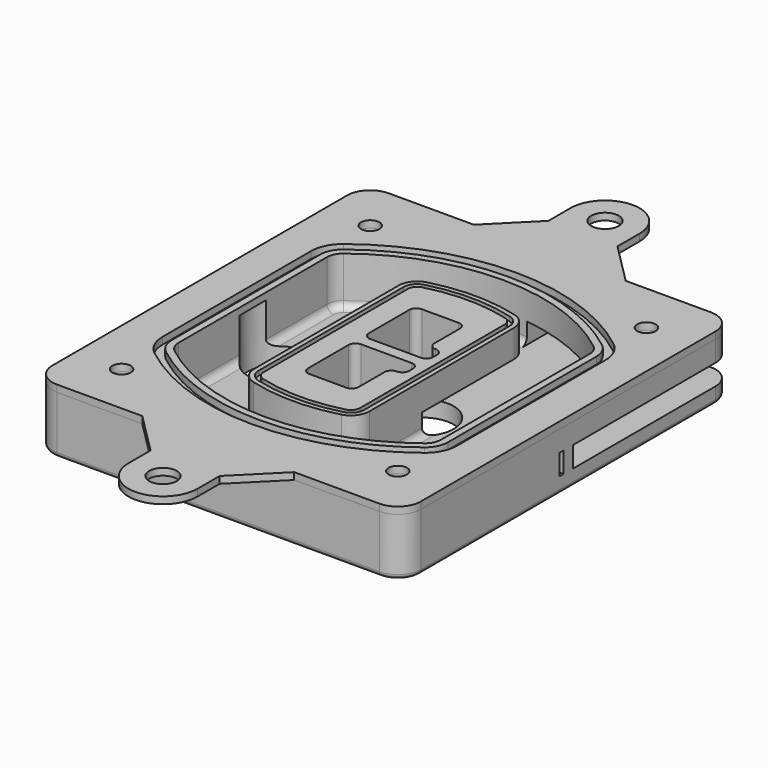
from build123d import *

# Parameters (mm, degrees)
F0_R      = 4
F1_DEPTH  = 25
F2_DEPTH  = 3
F3_DEPTH  = 18
F6_DEPTH  = 21
F7_DEPTH  = 2
F8_DEPTH  = 16
F9_DEPTH  = 25
F4_R      = 6
F4_R_2    = 4
F10_DEPTH = 6
F12_DEPTH = 9
F13_R     = 3
F14_R     = 2
F0_R_2    = 6
F15_DEPTH = 3
F17_DEPTH = 3


with BuildPart() as f1:
    # F0 (on Top) → F1 (new body)
    with BuildSketch(Plane.XY):
        with BuildLine():
            ThreePointArc((-80, -80), (-77.0710678119, -87.0710678119), (-70, -90))
            Line((-70, -90), (-33, -90))
            Line((-33, -90), (33, -90))
            Line((33, -90), (70, -90))
            ThreePointArc((70, -90), (77.0710678119, -87.0710678119), (80, -80))
            Line((80, -80), (80, 80))
            ThreePointArc((80, 80), (77.0710678119, 87.0710678119), (70, 90))
            Line((70, 90), (33, 90))
            Line((33, 90), (-33, 90))
            Line((-33, 90), (-70, 90))
            ThreePointArc((-70, 90), (-77.0710678119, 87.0710678119), (-80, 80))
            Line((-80, 80), (-80, -80))
        make_face()
        with Locations((-60, -67.5)):
            Circle(F0_R, mode=Mode.SUBTRACT)
        with Locations((60, -67.5)):
            Circle(F0_R, mode=Mode.SUBTRACT)
        with Locations((-60, 67.5)):
            Circle(F0_R, mode=Mode.SUBTRACT)
        with BuildLine():
            ThreePointArc((-64, 40.2934422872), (-62.5820384798, 46.4328484224), (-58.6153846154, 51.3286200352))
            ThreePointArc((-58.6153846154, 51.3286200352), (0, 71.5), (58.6153846154, 51.3286200352))
            ThreePointArc((58.6153846154, 51.3286200352), (62.5820384798, 46.4328484224), (64, 40.2934422872))
            Line((64, 40.2934422872), (64, -40.2934422872))
            ThreePointArc((64, -40.2934422872), (62.5820384798, -46.4328484224), (58.6153846154, -51.3286200352))
            ThreePointArc((58.6153846154, -51.3286200352), (0, -71.5), (-58.6153846154, -51.3286200352))
            ThreePointArc((-58.6153846154, -51.3286200352), (-62.5820384798, -46.4328484224), (-64, -40.2934422872))
            Line((-64, -40.2934422872), (-64, 40.2934422872))
        make_face(mode=Mode.SUBTRACT)
        with Locations((60, 67.5)):
            Circle(F0_R, mode=Mode.SUBTRACT)
        with BuildLine():
            ThreePointArc((58.6153846154, 51.3286200352), (0, 71.5), (-58.6153846154, 51.3286200352))
            ThreePointArc((-58.6153846154, 51.3286200352), (-62.5820384798, 46.4328484224), (-64, 40.2934422872))
            Line((-64, 40.2934422872), (-64, -40.2934422872))
            ThreePointArc((-64, -40.2934422872), (-62.5820384798, -46.4328484224), (-58.6153846154, -51.3286200352))
            ThreePointArc((-58.6153846154, -51.3286200352), (0, -71.5), (58.6153846154, -51.3286200352))
            ThreePointArc((58.6153846154, -51.3286200352), (62.5820384798, -46.4328484224), (64, -40.2934422872))
            Line((64, -40.2934422872), (64, 40.2934422872))
            ThreePointArc((64, 40.2934422872), (62.5820384798, 46.4328484224), (58.6153846154, 51.3286200352))
        make_face()
        with BuildLine():
            Line((-60, -40.2934422872), (-60, 40.2934422872))
            ThreePointArc((-60, 40.2934422872), (-58.9871703427, 44.6787323838), (-56.1538461538, 48.1757121072))
            ThreePointArc((-56.1538461538, 48.1757121072), (0, 67.5), (56.1538461538, 48.1757121072))
            ThreePointArc((56.1538461538, 48.1757121072), (58.9871703427, 44.6787323838), (60, 40.2934422872))
            Line((60, 40.2934422872), (60, -40.2934422872))
            ThreePointArc((60, -40.2934422872), (58.9871703427, -44.6787323838), (56.1538461538, -48.1757121072))
            ThreePointArc((56.1538461538, -48.1757121072), (0, -67.5), (-56.1538461538, -48.1757121072))
            ThreePointArc((-56.1538461538, -48.1757121072), (-58.9871703427, -44.6787323838), (-60, -40.2934422872))
        make_face(mode=Mode.SUBTRACT)
        with BuildLine():
            ThreePointArc((-56.1538461538, 48.1757121072), (-58.9871703427, 44.6787323838), (-60, 40.2934422872))
            Line((-60, 40.2934422872), (-60, -40.2934422872))
            ThreePointArc((-60, -40.2934422872), (-58.9871703427, -44.6787323838), (-56.1538461538, -48.1757121072))
            ThreePointArc((-56.1538461538, -48.1757121072), (0, -67.5), (56.1538461538, -48.1757121072))
            ThreePointArc((56.1538461538, -48.1757121072), (58.9871703427, -44.6787323838), (60, -40.2934422872))
            Line((60, -40.2934422872), (60, 40.2934422872))
            ThreePointArc((60, 40.2934422872), (58.9871703427, 44.6787323838), (56.1538461538, 48.1757121072))
            ThreePointArc((56.1538461538, 48.1757121072), (0, 67.5), (-56.1538461538, 48.1757121072))
        make_face()
        with BuildLine():
            ThreePointArc((54.3076923077, 45.8110311612), (56.2910192399, 43.3631453548), (57, 40.2934422872))
            Line((57, 40.2934422872), (57, -40.2934422872))
            ThreePointArc((57, -40.2934422872), (56.2910192399, -43.3631453548), (54.3076923077, -45.8110311612))
            ThreePointArc((54.3076923077, -45.8110311612), (0, -64.5), (-54.3076923077, -45.8110311612))
            ThreePointArc((-54.3076923077, -45.8110311612), (-56.2910192399, -43.3631453548), (-57, -40.2934422872))
            Line((-57, -40.2934422872), (-57, 40.2934422872))
            ThreePointArc((-57, 40.2934422872), (-56.2910192399, 43.3631453548), (-54.3076923077, 45.8110311612))
            ThreePointArc((-54.3076923077, 45.8110311612), (0, 64.5), (54.3076923077, 45.8110311612))
        make_face(mode=Mode.SUBTRACT)
        with BuildLine():
            Line((57, -40.2934422872), (57, 40.2934422872))
            ThreePointArc((57, 40.2934422872), (56.2910192399, 43.3631453548), (54.3076923077, 45.8110311612))
            ThreePointArc((54.3076923077, 45.8110311612), (0, 64.5), (-54.3076923077, 45.8110311612))
            ThreePointArc((-54.3076923077, 45.8110311612), (-56.2910192399, 43.3631453548), (-57, 40.2934422872))
            Line((-57, 40.2934422872), (-57, -40.2934422872))
            ThreePointArc((-57, -40.2934422872), (-56.2910192399, -43.3631453548), (-54.3076923077, -45.8110311612))
            ThreePointArc((-54.3076923077, -45.8110311612), (0, -64.5), (54.3076923077, -45.8110311612))
            ThreePointArc((54.3076923077, -45.8110311612), (56.2910192399, -43.3631453548), (57, -40.2934422872))
        make_face()
    extrude(amount=-F1_DEPTH)

    # F0 (on Top) → F2 (join)
    with BuildSketch(Plane.XY):
        with BuildLine():
            ThreePointArc((-56.1538461538, 48.1757121072), (-58.9871703427, 44.6787323838), (-60, 40.2934422872))
            Line((-60, 40.2934422872), (-60, -40.2934422872))
            ThreePointArc((-60, -40.2934422872), (-58.9871703427, -44.6787323838), (-56.1538461538, -48.1757121072))
            ThreePointArc((-56.1538461538, -48.1757121072), (0, -67.5), (56.1538461538, -48.1757121072))
            ThreePointArc((56.1538461538, -48.1757121072), (58.9871703427, -44.6787323838), (60, -40.2934422872))
            Line((60, -40.2934422872), (60, 40.2934422872))
            ThreePointArc((60, 40.2934422872), (58.9871703427, 44.6787323838), (56.1538461538, 48.1757121072))
            ThreePointArc((56.1538461538, 48.1757121072), (0, 67.5), (-56.1538461538, 48.1757121072))
        make_face()
        with BuildLine():
            ThreePointArc((54.3076923077, 45.8110311612), (56.2910192399, 43.3631453548), (57, 40.2934422872))
            Line((57, 40.2934422872), (57, -40.2934422872))
            ThreePointArc((57, -40.2934422872), (56.2910192399, -43.3631453548), (54.3076923077, -45.8110311612))
            ThreePointArc((54.3076923077, -45.8110311612), (0, -64.5), (-54.3076923077, -45.8110311612))
            ThreePointArc((-54.3076923077, -45.8110311612), (-56.2910192399, -43.3631453548), (-57, -40.2934422872))
            Line((-57, -40.2934422872), (-57, 40.2934422872))
            ThreePointArc((-57, 40.2934422872), (-56.2910192399, 43.3631453548), (-54.3076923077, 45.8110311612))
            ThreePointArc((-54.3076923077, 45.8110311612), (0, 64.5), (54.3076923077, 45.8110311612))
        make_face(mode=Mode.SUBTRACT)
    extrude(amount=F2_DEPTH)

    # F0 (on Top) → F3 (cut)
    with BuildSketch(Plane.XY):
        with BuildLine():
            Line((57, -40.2934422872), (57, 40.2934422872))
            ThreePointArc((57, 40.2934422872), (56.2910192399, 43.3631453548), (54.3076923077, 45.8110311612))
            ThreePointArc((54.3076923077, 45.8110311612), (0, 64.5), (-54.3076923077, 45.8110311612))
            ThreePointArc((-54.3076923077, 45.8110311612), (-56.2910192399, 43.3631453548), (-57, 40.2934422872))
            Line((-57, 40.2934422872), (-57, -40.2934422872))
            ThreePointArc((-57, -40.2934422872), (-56.2910192399, -43.3631453548), (-54.3076923077, -45.8110311612))
            ThreePointArc((-54.3076923077, -45.8110311612), (0, -64.5), (54.3076923077, -45.8110311612))
            ThreePointArc((54.3076923077, -45.8110311612), (56.2910192399, -43.3631453548), (57, -40.2934422872))
        make_face()
    extrude(amount=-F3_DEPTH, mode=Mode.SUBTRACT)

    # F5 (on face) → F6 (join, through all)
    with BuildSketch(Plane.XY.offset(3)):
        with BuildLine():
            ThreePointArc((-25, -39.2465276821), (-23.3511545998, -44.1109737193), (-19.0842911877, -46.9702398883))
            ThreePointArc((-19.0842911877, -46.9702398883), (0, -49.5), (19.0842911877, -46.9702398883))
            ThreePointArc((19.0842911877, -46.9702398883), (23.3511545998, -44.1109737193), (25, -39.2465276821))
            Line((25, -39.2465276821), (25, 39.2465276821))
            ThreePointArc((25, 39.2465276821), (23.3511545998, 44.1109737193), (19.0842911877, 46.9702398883))
            ThreePointArc((19.0842911877, 46.9702398883), (0, 49.5), (-19.0842911877, 46.9702398883))
            ThreePointArc((-19.0842911877, 46.9702398883), (-23.3511545998, 44.1109737193), (-25, 39.2465276821))
            Line((-25, 39.2465276821), (-25, -39.2465276821))
        make_face()
        with BuildLine():
            ThreePointArc((18.5632183908, 45.0393118368), (21.7633659499, 42.89486221), (23, 39.2465276821))
            Line((23, 39.2465276821), (23, -39.2465276821))
            ThreePointArc((23, -39.2465276821), (21.7633659499, -42.89486221), (18.5632183908, -45.0393118368))
            ThreePointArc((18.5632183908, -45.0393118368), (0, -47.5), (-18.5632183908, -45.0393118368))
            ThreePointArc((-18.5632183908, -45.0393118368), (-21.7633659499, -42.89486221), (-23, -39.2465276821))
            Line((-23, -39.2465276821), (-23, 39.2465276821))
            ThreePointArc((-23, 39.2465276821), (-21.7633659499, 42.89486221), (-18.5632183908, 45.0393118368))
            ThreePointArc((-18.5632183908, 45.0393118368), (0, 47.5), (18.5632183908, 45.0393118368))
        make_face(mode=Mode.SUBTRACT)
        with BuildLine():
            Line((23, -39.2465276821), (23, 39.2465276821))
            ThreePointArc((23, 39.2465276821), (21.7633659499, 42.89486221), (18.5632183908, 45.0393118368))
            ThreePointArc((18.5632183908, 45.0393118368), (0, 47.5), (-18.5632183908, 45.0393118368))
            ThreePointArc((-18.5632183908, 45.0393118368), (-21.7633659499, 42.89486221), (-23, 39.2465276821))
            Line((-23, 39.2465276821), (-23, -39.2465276821))
            ThreePointArc((-23, -39.2465276821), (-21.7633659499, -42.89486221), (-18.5632183908, -45.0393118368))
            ThreePointArc((-18.5632183908, -45.0393118368), (0, -47.5), (18.5632183908, -45.0393118368))
            ThreePointArc((18.5632183908, -45.0393118368), (21.7633659499, -42.89486221), (23, -39.2465276821))
        make_face()
        with BuildLine():
            ThreePointArc((18.0421455939, 43.1083837852), (20.1755772999, 41.6787507007), (21, 39.2465276821))
            Line((21, 39.2465276821), (21, -39.2465276821))
            ThreePointArc((21, -39.2465276821), (20.1755772999, -41.6787507007), (18.0421455939, -43.1083837852))
            ThreePointArc((18.0421455939, -43.1083837852), (0, -45.5), (-18.0421455939, -43.1083837852))
            ThreePointArc((-18.0421455939, -43.1083837852), (-20.1755772999, -41.6787507007), (-21, -39.2465276821))
            Line((-21, -39.2465276821), (-21, 39.2465276821))
            ThreePointArc((-21, 39.2465276821), (-20.1755772999, 41.6787507007), (-18.0421455939, 43.1083837852))
            ThreePointArc((-18.0421455939, 43.1083837852), (0, 45.5), (18.0421455939, 43.1083837852))
        make_face(mode=Mode.SUBTRACT)
        with BuildLine():
            Line((21, -39.2465276821), (21, 39.2465276821))
            ThreePointArc((21, 39.2465276821), (20.1755772999, 41.6787507007), (18.0421455939, 43.1083837852))
            ThreePointArc((18.0421455939, 43.1083837852), (0, 45.5), (-18.0421455939, 43.1083837852))
            ThreePointArc((-18.0421455939, 43.1083837852), (-20.1755772999, 41.6787507007), (-21, 39.2465276821))
            Line((-21, 39.2465276821), (-21, -39.2465276821))
            ThreePointArc((-21, -39.2465276821), (-20.1755772999, -41.6787507007), (-18.0421455939, -43.1083837852))
            ThreePointArc((-18.0421455939, -43.1083837852), (0, -45.5), (18.0421455939, -43.1083837852))
            ThreePointArc((18.0421455939, -43.1083837852), (20.1755772999, -41.6787507007), (21, -39.2465276821))
        make_face()
        with BuildLine():
            Line((-8, -2.5), (14, -2.5))
            ThreePointArc((14, -2.5), (16.1213203436, -3.3786796564), (17, -5.5))
            Line((17, -5.5), (17, -7.5))
            ThreePointArc((17, -7.5), (16.1213203436, -9.6213203436), (14, -10.5))
            ThreePointArc((14, -10.5), (11.8786796564, -11.3786796564), (11, -13.5))
            Line((11, -13.5), (11, -27.5))
            ThreePointArc((11, -27.5), (10.1213203436, -29.6213203436), (8, -30.5))
            Line((8, -30.5), (-8, -30.5))
            ThreePointArc((-8, -30.5), (-10.1213203436, -29.6213203436), (-11, -27.5))
            Line((-11, -27.5), (-11, -5.5))
            ThreePointArc((-11, -5.5), (-10.1213203436, -3.3786796564), (-8, -2.5))
        make_face(mode=Mode.SUBTRACT)
        with BuildLine():
            ThreePointArc((-8, 2.5), (-10.1213203436, 3.3786796564), (-11, 5.5))
            Line((-11, 5.5), (-11, 27.5))
            ThreePointArc((-11, 27.5), (-10.1213203436, 29.6213203436), (-8, 30.5))
            Line((-8, 30.5), (8, 30.5))
            ThreePointArc((8, 30.5), (10.1213203436, 29.6213203436), (11, 27.5))
            Line((11, 27.5), (11, 13.5))
            ThreePointArc((11, 13.5), (11.8786796564, 11.3786796564), (14, 10.5))
            ThreePointArc((14, 10.5), (16.1213203436, 9.6213203436), (17, 7.5))
            Line((17, 7.5), (17, 5.5))
            ThreePointArc((17, 5.5), (16.1213203436, 3.3786796564), (14, 2.5))
            Line((14, 2.5), (-8, 2.5))
        make_face(mode=Mode.SUBTRACT)
    extrude(amount=-F6_DEPTH)

    # F5 (on face) → F7 (cut)
    with BuildSketch(Plane.XY.offset(3)):
        with BuildLine():
            Line((23, -39.2465276821), (23, 39.2465276821))
            ThreePointArc((23, 39.2465276821), (21.7633659499, 42.89486221), (18.5632183908, 45.0393118368))
            ThreePointArc((18.5632183908, 45.0393118368), (0, 47.5), (-18.5632183908, 45.0393118368))
            ThreePointArc((-18.5632183908, 45.0393118368), (-21.7633659499, 42.89486221), (-23, 39.2465276821))
            Line((-23, 39.2465276821), (-23, -39.2465276821))
            ThreePointArc((-23, -39.2465276821), (-21.7633659499, -42.89486221), (-18.5632183908, -45.0393118368))
            ThreePointArc((-18.5632183908, -45.0393118368), (0, -47.5), (18.5632183908, -45.0393118368))
            ThreePointArc((18.5632183908, -45.0393118368), (21.7633659499, -42.89486221), (23, -39.2465276821))
        make_face()
        with BuildLine():
            ThreePointArc((18.0421455939, 43.1083837852), (20.1755772999, 41.6787507007), (21, 39.2465276821))
            Line((21, 39.2465276821), (21, -39.2465276821))
            ThreePointArc((21, -39.2465276821), (20.1755772999, -41.6787507007), (18.0421455939, -43.1083837852))
            ThreePointArc((18.0421455939, -43.1083837852), (0, -45.5), (-18.0421455939, -43.1083837852))
            ThreePointArc((-18.0421455939, -43.1083837852), (-20.1755772999, -41.6787507007), (-21, -39.2465276821))
            Line((-21, -39.2465276821), (-21, 39.2465276821))
            ThreePointArc((-21, 39.2465276821), (-20.1755772999, 41.6787507007), (-18.0421455939, 43.1083837852))
            ThreePointArc((-18.0421455939, 43.1083837852), (0, 45.5), (18.0421455939, 43.1083837852))
        make_face(mode=Mode.SUBTRACT)
    extrude(amount=-F7_DEPTH, mode=Mode.SUBTRACT)

    # F4 (on face) → F8 (cut)
    with BuildSketch(Plane(origin=(0, 0, -25), x_dir=(1, 0, 0), z_dir=(0, 0, -1))):
        with BuildLine():
            Line((3.28842436, 0), (30.224982775, 0))
            ThreePointArc((30.224982775, 0), (16.7567035675, 13.4682792075), (3.28842436, 0))
        make_face()
        with BuildLine():
            ThreePointArc((3.28842436, 0), (16.7567035675, -13.4682792075), (30.224982775, 0))
            Line((30.224982775, 0), (3.28842436, 0))
        make_face()
    extrude(amount=-F8_DEPTH, mode=Mode.SUBTRACT)

    # F4 (on face) → F9 (cut)
    with BuildSketch(Plane(origin=(0, 0, -25), x_dir=(1, 0, 0), z_dir=(0, 0, -1))):
        with BuildLine():
            Line((-59.0318229325, 0), (-32.0952645175, 0))
            ThreePointArc((-32.0952645175, 0), (-45.563543725, 13.4682792075), (-59.0318229325, 0))
        make_face()
        with BuildLine():
            ThreePointArc((-59.0318229325, 0), (-45.563543725, -13.4682792075), (-32.0952645175, 0))
            Line((-32.0952645175, 0), (-59.0318229325, 0))
        make_face()
    extrude(amount=-F9_DEPTH, mode=Mode.SUBTRACT)

    # F4 (on face) → F10 (cut)
    with BuildSketch(Plane(origin=(0, 0, -25), x_dir=(1, 0, 0), z_dir=(0, 0, -1))):
        with Locations((60, -67.5)):
            Circle(F4_R)
        with Locations((60, -67.5)):
            Circle(F4_R_2, mode=Mode.SUBTRACT)
        with Locations((-60, -67.5)):
            Circle(F4_R)
        with Locations((-60, -67.5)):
            Circle(F4_R_2, mode=Mode.SUBTRACT)
        with Locations((-60, 67.5)):
            Circle(F4_R)
        with Locations((-60, 67.5)):
            Circle(F4_R_2, mode=Mode.SUBTRACT)
        with Locations((60, 67.5)):
            Circle(F4_R)
        with Locations((60, 67.5)):
            Circle(F4_R_2, mode=Mode.SUBTRACT)
    extrude(amount=-F10_DEPTH, mode=Mode.SUBTRACT)

    # F11 (on face) → F12 (cut, through all)
    with BuildSketch(Plane(origin=(0, 0, -9), x_dir=(1, 0, 0), z_dir=(0, 0, -1))):
        with BuildLine():
            Line((11, -13.5), (11, -88.1870589921))
            ThreePointArc((11, -88.1870589921), (97.0977373733, -83.5977373733), (92.5084157545, 2.5))
            Line((92.5084157545, 2.5), (84.3581178167, 2.5))
            ThreePointArc((84.3581178167, 2.5), (88.518366543, 0.1387176755), (92.5084157545, -2.5))
            Line((92.5084157545, -2.5), (25, -2.5))
            Line((25, -2.5), (25, -10.6509440304))
            ThreePointArc((25, -10.6509440304), (18.3539136316, -13.3732368865), (11.2536447004, -12.2927168648))
            ThreePointArc((11.2536447004, -12.2927168648), (11.0640958889, -12.8831798879), (11, -13.5))
        make_face()
        with BuildLine():
            Line((11, -2.5), (11, -13.5))
            ThreePointArc((11, -13.5), (11.0640958889, -12.8831798879), (11.2536447004, -12.2927168648))
            ThreePointArc((11.2536447004, -12.2927168648), (12.3601599782, -10.9878446101), (14, -10.5))
            ThreePointArc((14, -10.5), (16.1213203436, -9.6213203436), (17, -7.5))
            Line((17, -7.5), (17, -5.5))
            ThreePointArc((17, -5.5), (16.1213203436, -3.3786796564), (14, -2.5))
            Line((14, -2.5), (11, -2.5))
        make_face()
        with BuildLine():
            Line((25, 2.5), (84.3581178167, 2.5))
            ThreePointArc((84.3581178167, 2.5), (54.981370865, 10.4428949133), (25, 5.2275097766))
            Line((25, 5.2275097766), (25, 2.5))
        make_face()
        with BuildLine():
            ThreePointArc((19.1502979378, 2.5), (14.9900492115, 0.1387176755), (11, -2.5))
            Line((11, -2.5), (14, -2.5))
            Line((14, -2.5), (25, -2.5))
            Line((25, -2.5), (25, 2.5))
            Line((25, 2.5), (19.1502979378, 2.5))
        make_face()
        with BuildLine():
            Line((25, 2.5), (25, 5.2275097766))
            ThreePointArc((25, 5.2275097766), (22.0438331728, 3.9309180122), (19.1502979378, 2.5))
            Line((19.1502979378, 2.5), (25, 2.5))
        make_face()
        with BuildLine():
            Line((11, 13.5), (11, 2.5))
            Line((11, 2.5), (14, 2.5))
            ThreePointArc((14, 2.5), (16.1213203436, 3.3786796564), (17, 5.5))
            Line((17, 5.5), (17, 7.5))
            ThreePointArc((17, 7.5), (16.1213203436, 9.6213203436), (14, 10.5))
            ThreePointArc((14, 10.5), (12.3601599782, 10.9878446101), (11.2536447004, 12.2927168648))
            ThreePointArc((11.2536447004, 12.2927168648), (11.0640958889, 12.8831798879), (11, 13.5))
        make_face()
    extrude(amount=F12_DEPTH, mode=Mode.SUBTRACT)

    # F13
    f13_edges = [f1.edges().sort_by_distance(p)[0] for p in [
        (-57, -23.703476, -18),
        (-57, 23.703476, -18),
        (25, -24.948736, -18),
        (57, -25.307233, -18),
        (-56.291019, 43.363145, -18),
        (-56.291019, -43.363145, -18),
        (0, -64.5, -18),
        (-23.449854, 61.327417, -18),
        (56.291019, -43.363145, -18),
        (-4.130458, 49.383452, -18),
        (-23.351155, 44.110974, -18),
        (-25, 0, -18),
        (-23.351155, -44.110974, -18),
        (0, -49.5, -18),
        (23.351155, -44.110974, -18),
    ]]
    fillet(f13_edges, radius=F13_R)

    # F14
    f14_edges = [f1.edges().sort_by_distance(p)[0] for p in [
        (0, -90, -25),
        (80, 0, -25),
        (0, 90, -25),
        (77.071068, 87.071068, -25),
        (-77.071068, 87.071068, -25),
        (-80, 0, -25),
        (77.071068, -87.071068, -25),
        (-77.071068, -87.071068, -25),
    ]]
    fillet(f14_edges, radius=F14_R)


with BuildPart() as f15:
    # F0 (on Top) → F15 (new body, through all)
    with BuildSketch(Plane.XY):
        with BuildLine():
            ThreePointArc((-80, -80), (-77.0710678119, -87.0710678119), (-70, -90))
            Line((-70, -90), (-33, -90))
            Line((-33, -90), (33, -90))
            Line((33, -90), (70, -90))
            ThreePointArc((70, -90), (77.0710678119, -87.0710678119), (80, -80))
            Line((80, -80), (80, 80))
            ThreePointArc((80, 80), (77.0710678119, 87.0710678119), (70, 90))
            Line((70, 90), (33, 90))
            Line((33, 90), (-33, 90))
            Line((-33, 90), (-70, 90))
            ThreePointArc((-70, 90), (-77.0710678119, 87.0710678119), (-80, 80))
            Line((-80, 80), (-80, -80))
        make_face()
        with Locations((-60, -67.5)):
            Circle(F0_R, mode=Mode.SUBTRACT)
        with Locations((60, -67.5)):
            Circle(F0_R, mode=Mode.SUBTRACT)
        with Locations((-60, 67.5)):
            Circle(F0_R, mode=Mode.SUBTRACT)
        with BuildLine():
            ThreePointArc((-64, 40.2934422872), (-62.5820384798, 46.4328484224), (-58.6153846154, 51.3286200352))
            ThreePointArc((-58.6153846154, 51.3286200352), (0, 71.5), (58.6153846154, 51.3286200352))
            ThreePointArc((58.6153846154, 51.3286200352), (62.5820384798, 46.4328484224), (64, 40.2934422872))
            Line((64, 40.2934422872), (64, -40.2934422872))
            ThreePointArc((64, -40.2934422872), (62.5820384798, -46.4328484224), (58.6153846154, -51.3286200352))
            ThreePointArc((58.6153846154, -51.3286200352), (0, -71.5), (-58.6153846154, -51.3286200352))
            ThreePointArc((-58.6153846154, -51.3286200352), (-62.5820384798, -46.4328484224), (-64, -40.2934422872))
            Line((-64, -40.2934422872), (-64, 40.2934422872))
        make_face(mode=Mode.SUBTRACT)
        with Locations((60, 67.5)):
            Circle(F0_R, mode=Mode.SUBTRACT)
        with BuildLine():
            Line((33, -90), (-33, -90))
            Line((-33, -90), (-15, -108))
            Line((-15, -108), (-15, -120))
            ThreePointArc((-15, -120), (0, -135), (15, -120))
            Line((15, -120), (15, -108))
            Line((15, -108), (33, -90))
        make_face()
        with Locations((0, -120)):
            Circle(F0_R_2, mode=Mode.SUBTRACT)
        with BuildLine():
            Line((-15, 108), (-33, 90))
            Line((-33, 90), (33, 90))
            Line((33, 90), (15, 108))
            Line((15, 108), (15, 120))
            ThreePointArc((15, 120), (0, 135), (-15, 120))
            Line((-15, 120), (-15, 108))
        make_face()
        with Locations((0, 120)):
            Circle(F0_R_2, mode=Mode.SUBTRACT)
    extrude(amount=F15_DEPTH)


with BuildPart() as f17:
    # F0 (on Top) → F17 (new body, through all)
    with BuildSketch(Plane.XY):
        with BuildLine():
            ThreePointArc((-80, -80), (-77.0710678119, -87.0710678119), (-70, -90))
            Line((-70, -90), (-33, -90))
            Line((-33, -90), (33, -90))
            Line((33, -90), (70, -90))
            ThreePointArc((70, -90), (77.0710678119, -87.0710678119), (80, -80))
            Line((80, -80), (80, 80))
            ThreePointArc((80, 80), (77.0710678119, 87.0710678119), (70, 90))
            Line((70, 90), (33, 90))
            Line((33, 90), (-33, 90))
            Line((-33, 90), (-70, 90))
            ThreePointArc((-70, 90), (-77.0710678119, 87.0710678119), (-80, 80))
            Line((-80, 80), (-80, -80))
        make_face()
        with Locations((-60, -67.5)):
            Circle(F0_R, mode=Mode.SUBTRACT)
        with Locations((60, -67.5)):
            Circle(F0_R, mode=Mode.SUBTRACT)
        with Locations((-60, 67.5)):
            Circle(F0_R, mode=Mode.SUBTRACT)
        with BuildLine():
            ThreePointArc((-64, 40.2934422872), (-62.5820384798, 46.4328484224), (-58.6153846154, 51.3286200352))
            ThreePointArc((-58.6153846154, 51.3286200352), (0, 71.5), (58.6153846154, 51.3286200352))
            ThreePointArc((58.6153846154, 51.3286200352), (62.5820384798, 46.4328484224), (64, 40.2934422872))
            Line((64, 40.2934422872), (64, -40.2934422872))
            ThreePointArc((64, -40.2934422872), (62.5820384798, -46.4328484224), (58.6153846154, -51.3286200352))
            ThreePointArc((58.6153846154, -51.3286200352), (0, -71.5), (-58.6153846154, -51.3286200352))
            ThreePointArc((-58.6153846154, -51.3286200352), (-62.5820384798, -46.4328484224), (-64, -40.2934422872))
            Line((-64, -40.2934422872), (-64, 40.2934422872))
        make_face(mode=Mode.SUBTRACT)
        with Locations((60, 67.5)):
            Circle(F0_R, mode=Mode.SUBTRACT)
        with BuildLine():
            Line((33, -90), (-33, -90))
            Line((-33, -90), (-15, -108))
            Line((-15, -108), (-15, -120))
            ThreePointArc((-15, -120), (0, -135), (15, -120))
            Line((15, -120), (15, -108))
            Line((15, -108), (33, -90))
        make_face()
        with Locations((0, -120)):
            Circle(F0_R_2, mode=Mode.SUBTRACT)
        with BuildLine():
            Line((-15, 108), (-33, 90))
            Line((-33, 90), (33, 90))
            Line((33, 90), (15, 108))
            Line((15, 108), (15, 120))
            ThreePointArc((15, 120), (0, 135), (-15, 120))
            Line((-15, 120), (-15, 108))
        make_face()
        with Locations((0, 120)):
            Circle(F0_R_2, mode=Mode.SUBTRACT)
    extrude(amount=F17_DEPTH)


solid = Compound([f1.part, f17.part])
